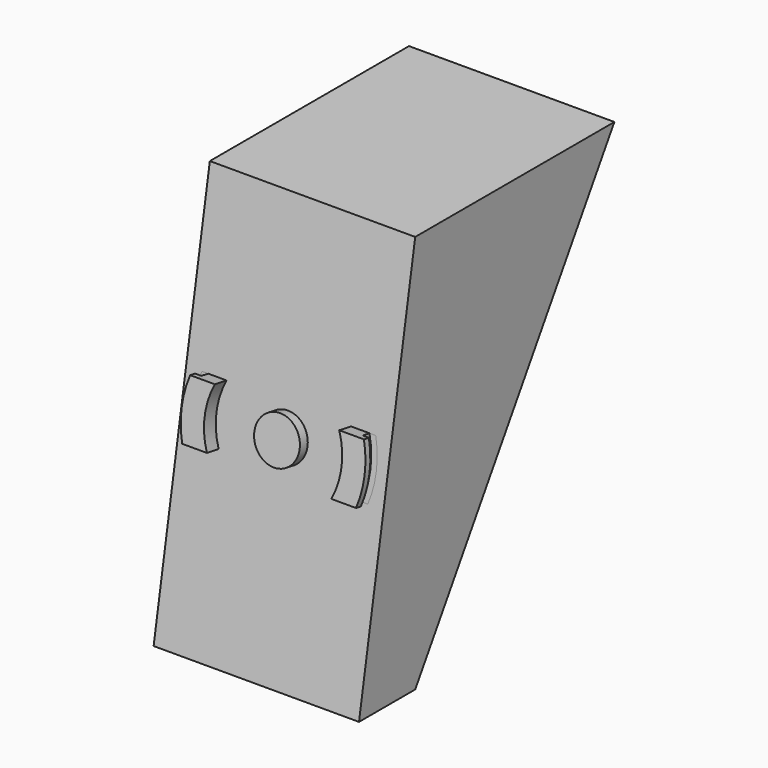
from build123d import *

# Parameters (mm, degrees)
F1_DEPTH = 41.91
F2_R     = 4.6355
F3_DEPTH = 2.032
F4_DEPTH = 3.048
F5_DEPTH = 1.778


with BuildPart() as f1:
    # F0 (on Right) → F1 (new body)
    with BuildSketch(Plane.YZ):
        Polygon((50.8, 0), (0, 0), (-14.3346570664, -81.2958800112), (0, -81.2958800112), align=None)
    extrude(amount=-F1_DEPTH)

    # F2 (on face) → F3 (join)
    with BuildSketch(Plane(origin=(0, 0, 0), x_dir=(1, 0, 0), z_dir=(0, -0.984807753, 0.1736481777))):
        with Locations((-20.955, -40.64)):
            Circle(F2_R)
    extrude(amount=F3_DEPTH)

    # F2 (on face) → F4 (join)
    with BuildSketch(Plane(origin=(0, 0, 0), x_dir=(1, 0, 0), z_dir=(0, -0.984807753, 0.1736481777))):
        with BuildLine():
            ThreePointArc((-8.2651640673, -34.798), (-6.985, -40.64), (-8.2651640673, -46.482))
            Line((-8.2651640673, -46.482), (-4.4986959724, -46.482))
            ThreePointArc((-4.4986959724, -46.482), (-3.4925, -40.64), (-4.4986959724, -34.798))
            Line((-4.4986959724, -34.798), (-8.2651640673, -34.798))
        make_face()
        with BuildLine():
            ThreePointArc((-4.4986959724, -34.798), (-3.4925, -40.64), (-4.4986959724, -46.482))
            Line((-4.4986959724, -46.482), (-3.2235985607, -46.482))
            ThreePointArc((-3.2235985607, -46.482), (-2.286, -40.64), (-3.2235985607, -34.798))
            Line((-3.2235985607, -34.798), (-4.4986959724, -34.798))
        make_face()
    extrude(amount=F4_DEPTH)

    # F2 (on face) → F5 (cut)
    with BuildSketch(Plane(origin=(0, 0, 0), x_dir=(1, 0, 0), z_dir=(0, -0.984807753, 0.1736481777))):
        with BuildLine():
            ThreePointArc((-4.4986959724, -34.798), (-3.4925, -40.64), (-4.4986959724, -46.482))
            Line((-4.4986959724, -46.482), (-3.2235985607, -46.482))
            ThreePointArc((-3.2235985607, -46.482), (-2.286, -40.64), (-3.2235985607, -34.798))
            Line((-3.2235985607, -34.798), (-4.4986959724, -34.798))
        make_face()
    extrude(amount=F5_DEPTH, mode=Mode.SUBTRACT)

    # F7: F1 across plane


with BuildPart() as f1_1:
    add(f1.part)
    add(f1.part.mirror(Plane(origin=(-20.955, 12.1551143112, -33.0624182644), x_dir=(0, 1, 0), z_dir=(1, 0, 0))))


solid = f1_1.part
